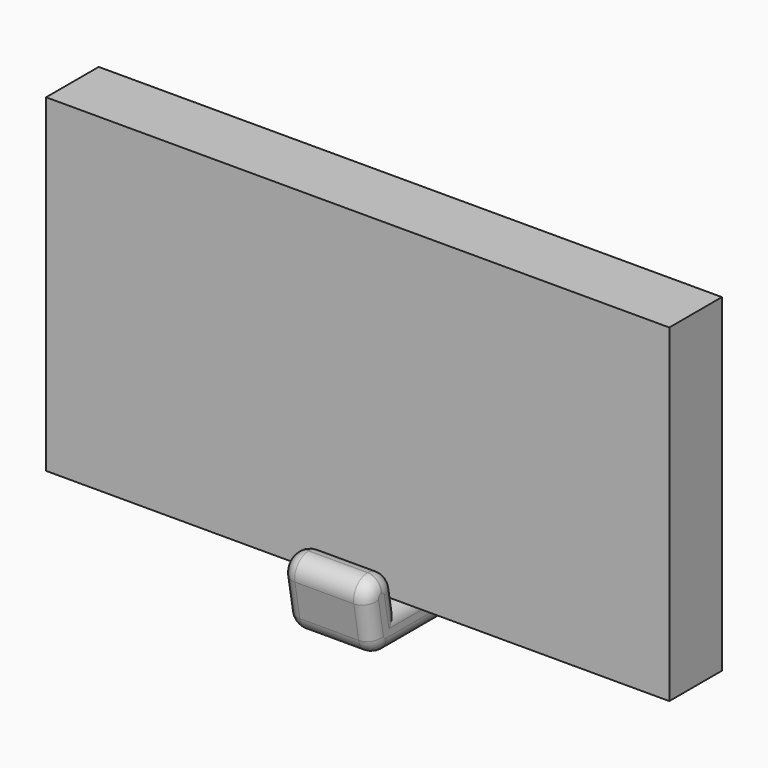
from build123d import *

# Parameters (mm, degrees)
F0_W          = 180
F0_H          = 95
F1_DEPTH      = 9.5
F3_W          = 10
F3_H          = 69.3333333333
F3_W_2        = 5
F3_H_2        = 10
F4_DEPTH      = 12.5
F5_T1_DEPTH   = 10.1542661189
F5_T3_DEPTH   = 65.3333333333
F5_T5_DEPTH   = 2
F5_T7_DEPTH   = 17
F5_T9_DEPTH   = 30.3474206258
F5_T11_DEPTH  = 70.3333333333
F5_T13_DEPTH  = 0.1519224699
F5_S17_W      = 4
F5_S17_H      = 4
F5_T18_DEPTH  = 4
F5_S23_W      = 4
F5_S23_H      = 4
F5_T24_DEPTH  = 4
F5_S29_W      = 4
F5_S29_H      = 4
F5_T30_DEPTH  = 4
F5_S35_W      = 4
F5_S35_H      = 4
F5_T36_DEPTH  = 4
F5_T42_DEPTH  = 31
F5_T47_DEPTH  = 31
F5_T50_ANGLE  = 100
F5_T52_ANGLE  = 80
F5_T54_ANGLE  = 90
F5_T56_ANGLE  = 80
F5_T60_DEPTH  = 15.958767963
F5_T63_ANGLE  = 100
F5_T65_ANGLE  = 80
F5_T67_ANGLE  = 90
F5_T69_ANGLE  = 80
F5_T73_DEPTH  = 15.958767963
F5_T79_DEPTH  = 75.3333333333
F5_T83_DEPTH  = 41
F5_T90_DEPTH  = 15.958767963
F5_T94_DEPTH  = 31
F5_T101_DEPTH = 75.3333333333
F5_T105_DEPTH = 41
F5_T112_DEPTH = 15.958767963
F5_T116_DEPTH = 31
F6_W          = 119.8909639199
F6_H          = 5
F7_DEPTH      = 5


# Not quite as in the source:
# - a fillet or chamfer that OpenCascade refuses, or shapes differently, is made with other operations: its cross-section is extruded or revolved along the edge and cut away or added


with BuildPart() as f1:
    # F0 (on Front) → F1 (new body, symmetric)
    with BuildSketch(Plane.XZ):
        Rectangle(F0_W, F0_H)
    extrude(amount=F1_DEPTH, both=True)


with BuildPart() as f4:
    # F3 (on Right) → F4 (new body, symmetric)
    with BuildSketch(Plane.YZ):
        with Locations((15.5, -13.8333333333)):
            Rectangle(F3_W, F3_H)
        with Locations((15.5, 10.8333333333)):
            Rectangle(F3_W_2, F3_H_2, mode=Mode.SUBTRACT)
        with BuildLine():
            Line((20.5, -53.5), (20.5, -48.5))
            Line((20.5, -48.5), (10.5, -48.5))
            Line((10.5, -48.5), (-10.5, -48.5))
            Line((-10.5, -48.5), (-8.7367301929, -58.5))
            Line((-8.7367301929, -58.5), (15.5, -58.5))
            ThreePointArc((15.5, -58.5), (19.0355339059, -57.0355339059), (20.5, -53.5))
        make_face()
        Polygon((-8.7367301929, -58.5), (-10.5, -48.5), (-10.5, -58.5), align=None)
        with BuildLine():
            Line((-10.5, -58.5), (-10.5, -48.5))
            Line((-10.5, -48.5), (-11.5347291979, -42.6317591117))
            ThreePointArc((-11.5347291979, -42.6317591117), (-13.2448299145, -39.6697777844), (-16.458767963, -38.5))
            Line((-16.458767963, -38.5), (-16.6106904328, -38.5))
            ThreePointArc((-16.6106904328, -38.5), (-20.4409126484, -40.2860619516), (-21.5347291979, -44.3682408883))
            Line((-21.5347291979, -44.3682408883), (-19.7714593908, -54.3682408883))
            ThreePointArc((-19.7714593908, -54.3682408883), (-18.0613586742, -57.3302222156), (-14.8474206258, -58.5))
            Line((-14.8474206258, -58.5), (-10.5, -58.5))
        make_face()
    extrude(amount=F4_DEPTH, both=True)

    # F5: fillet of radius 4 on 10 edges, made by hand

    # F5_s2 → F5_t1 (cut)
    with BuildSketch(Plane(origin=(0, 6.9380645139, -39.3477191408), x_dir=(1, 0, 0), z_dir=(0, 0.1736481777, -0.984807753))):
        with BuildLine():
            ThreePointArc((-8.5, 28.9120324497), (-11.3284271247, 27.7404595744), (-12.5, 24.9120324497))
            Line((-12.5, 24.9120324497), (-12.5, 28.9120324497))
            Line((-12.5, 28.9120324497), (-8.5, 28.9120324497))
        make_face()
        with BuildLine():
            ThreePointArc((8.5, 28.9120324497), (11.3284271247, 27.7404595744), (12.5, 24.9120324497))
            Line((12.5, 24.9120324497), (12.5, 28.9120324497))
            Line((12.5, 28.9120324497), (8.5, 28.9120324497))
        make_face()
    extrude(amount=F5_T1_DEPTH, mode=Mode.SUBTRACT)

    # F5_s4 → F5_t3 (cut)
    with BuildSketch(Plane.XY.offset(-48.5)):
        with BuildLine():
            ThreePointArc((8.5, 10.5), (11.3284271247, 11.6715728753), (12.5, 14.5))
            Line((12.5, 14.5), (12.5, 10.5))
            Line((12.5, 10.5), (8.5, 10.5))
        make_face()
        with BuildLine():
            ThreePointArc((-8.5, 10.5), (-11.3284271247, 11.6715728753), (-12.5, 14.5))
            Line((-12.5, 14.5), (-12.5, 10.5))
            Line((-12.5, 10.5), (-8.5, 10.5))
        make_face()
    extrude(amount=F5_T3_DEPTH, mode=Mode.SUBTRACT)

    # F5_s6 → F5_t5 (cut)
    with BuildSketch(Plane.XZ.offset(-16.5)):
        with BuildLine():
            ThreePointArc((-8.5, 20.8333333333), (-11.3284271247, 19.6617604581), (-12.5, 16.8333333333))
            Line((-12.5, 16.8333333333), (-12.5, 20.8333333333))
            Line((-12.5, 20.8333333333), (-8.5, 20.8333333333))
        make_face()
        with BuildLine():
            ThreePointArc((8.5, 20.8333333333), (11.3284271247, 19.6617604581), (12.5, 16.8333333333))
            Line((12.5, 16.8333333333), (12.5, 20.8333333333))
            Line((12.5, 20.8333333333), (8.5, 20.8333333333))
        make_face()
    extrude(amount=F5_T5_DEPTH, mode=Mode.SUBTRACT)

    # F5_s8 → F5_t7 (cut)
    with BuildSketch(Plane.YZ.offset(-8.5)):
        with BuildLine():
            ThreePointArc((10.5, 16.8333333333), (11.6715728753, 19.6617604581), (14.5, 20.8333333333))
            Line((14.5, 20.8333333333), (10.5, 20.8333333333))
            Line((10.5, 20.8333333333), (10.5, 16.8333333333))
        make_face()
        with BuildLine():
            ThreePointArc((16.5, 20.8333333333), (19.3284271247, 19.6617604581), (20.5, 16.8333333333))
            Line((20.5, 16.8333333333), (20.5, 20.8333333333))
            Line((20.5, 20.8333333333), (16.5, 20.8333333333))
        make_face()
    extrude(amount=F5_T7_DEPTH, mode=Mode.SUBTRACT)

    # F5_s10 → F5_t9 (cut)
    with BuildSketch(Plane.XZ.offset(-15.5)):
        with BuildLine():
            ThreePointArc((8.5, -58.5), (11.3284271247, -57.3284271247), (12.5, -54.5))
            Line((12.5, -54.5), (12.5, -58.5))
            Line((12.5, -58.5), (8.5, -58.5))
        make_face()
        with BuildLine():
            ThreePointArc((-8.5, -58.5), (-11.3284271247, -57.3284271247), (-12.5, -54.5))
            Line((-12.5, -54.5), (-12.5, -58.5))
            Line((-12.5, -58.5), (-8.5, -58.5))
        make_face()
    extrude(amount=F5_T9_DEPTH, mode=Mode.SUBTRACT)

    # F5_s12 → F5_t11 (cut)
    with BuildSketch(Plane.XY.offset(-53.5)):
        with BuildLine():
            ThreePointArc((8.5, 20.5), (11.3284271247, 19.3284271247), (12.5, 16.5))
            Line((12.5, 16.5), (12.5, 20.5))
            Line((12.5, 20.5), (8.5, 20.5))
        make_face()
        with BuildLine():
            ThreePointArc((-8.5, 20.5), (-11.3284271247, 19.3284271247), (-12.5, 16.5))
            Line((-12.5, 16.5), (-12.5, 20.5))
            Line((-12.5, 20.5), (-8.5, 20.5))
        make_face()
    extrude(amount=F5_T11_DEPTH, mode=Mode.SUBTRACT)

    # F5_s14 → F5_t13 (cut)
    with BuildSketch(Plane.XZ.offset(16.458767963)):
        with BuildLine():
            ThreePointArc((8.5, -38.5), (11.3284271247, -39.6715728753), (12.5, -42.5))
            Line((12.5, -42.5), (12.5, -38.5))
            Line((12.5, -38.5), (8.5, -38.5))
        make_face()
        with BuildLine():
            ThreePointArc((-8.5, -38.5), (-11.3284271247, -39.6715728753), (-12.5, -42.5))
            Line((-12.5, -42.5), (-12.5, -38.5))
            Line((-12.5, -38.5), (-8.5, -38.5))
        make_face()
    extrude(amount=F5_T13_DEPTH, mode=Mode.SUBTRACT)


with BuildPart() as f5_tool16:
    # F5_s17 → F5_t18 (new body)
    with BuildSketch(Plane.XZ.offset(-14.5)):
        with Locations((10.5, 18.8333333333)):
            Rectangle(F5_S17_W, F5_S17_H)
    extrude(amount=F5_T18_DEPTH)

    # F5_s19 → F5_t20 (revolve, cut)
    with BuildSketch(Plane(origin=(8.5, 14.5, 16.8333333333), x_dir=(-0.7071067812, 0, -0.7071067812), z_dir=(-0.7071067812, 0, 0.7071067812))):
        with BuildLine():
            ThreePointArc((0, -4), (4, 0), (0, 4))
            Line((0, 4), (0, -4))
        make_face()
    revolve(axis=Axis((8.5, 14.5, 16.8333333333), (0, -1, 0)), mode=Mode.SUBTRACT)


with BuildPart() as f4_1:
    add(f4.part)

    # F5_t15: cut F5_tool16
    add(f5_tool16.part, mode=Mode.SUBTRACT)


with BuildPart() as f5_tool22:
    # F5_s23 → F5_t24 (new body)
    with BuildSketch(Plane.XZ.offset(-14.5)):
        with Locations((-10.5, 18.8333333333)):
            Rectangle(F5_S23_W, F5_S23_H)
    extrude(amount=F5_T24_DEPTH)

    # F5_s25 → F5_t26 (revolve, cut)
    with BuildSketch(Plane(origin=(-8.5, 14.5, 16.8333333333), x_dir=(0.7071067812, 0, -0.7071067812), z_dir=(-0.7071067812, 0, -0.7071067812))):
        with BuildLine():
            ThreePointArc((0, -4), (4, 0), (0, 4))
            Line((0, 4), (0, -4))
        make_face()
    revolve(axis=Axis((-8.5, 14.5, 16.8333333333), (0, -1, 0)), mode=Mode.SUBTRACT)


with BuildPart() as f4_2:
    add(f4_1.part)

    # F5_t21: cut F5_tool22
    add(f5_tool22.part, mode=Mode.SUBTRACT)


with BuildPart() as f5_tool28:
    # F5_s29 → F5_t30 (new body)
    with BuildSketch(Plane.XY.offset(16.8333333333)):
        with Locations((-10.5, 18.5)):
            Rectangle(F5_S29_W, F5_S29_H)
    extrude(amount=F5_T30_DEPTH)

    # F5_s31 → F5_t32 (revolve, cut)
    with BuildSketch(Plane(origin=(-8.5, 16.5, 16.8333333333), x_dir=(0.7071067812, -0.7071067812, 0), z_dir=(-0.7071067812, -0.7071067812, 0))):
        with BuildLine():
            ThreePointArc((0, -4), (4, 0), (0, 4))
            Line((0, 4), (0, -4))
        make_face()
    revolve(axis=Axis((-8.5, 16.5, 16.8333333333), (0, 0, 1)), mode=Mode.SUBTRACT)


with BuildPart() as f4_3:
    add(f4_2.part)

    # F5_t27: cut F5_tool28
    add(f5_tool28.part, mode=Mode.SUBTRACT)


with BuildPart() as f5_tool34:
    # F5_s35 → F5_t36 (new body)
    with BuildSketch(Plane.XY.offset(16.8333333333)):
        with Locations((10.5, 18.5)):
            Rectangle(F5_S35_W, F5_S35_H)
    extrude(amount=F5_T36_DEPTH)

    # F5_s37 → F5_t38 (revolve, cut)
    with BuildSketch(Plane(origin=(8.5, 16.5, 16.8333333333), x_dir=(-0.7071067812, -0.7071067812, 0), z_dir=(-0.7071067812, 0.7071067812, 0))):
        with BuildLine():
            ThreePointArc((0, -4), (4, 0), (0, 4))
            Line((0, 4), (0, -4))
        make_face()
    revolve(axis=Axis((8.5, 16.5, 16.8333333333), (0, 0, 1)), mode=Mode.SUBTRACT)


with BuildPart() as f4_4:
    add(f4_3.part)

    # F5_t33: cut F5_tool34
    add(f5_tool34.part, mode=Mode.SUBTRACT)


with BuildPart() as f5_tool40:
    # F5_s41 → F5_t42 (new body)
    with BuildSketch(Plane.XZ.offset(-10.5)):
        with BuildLine():
            ThreePointArc((12.5, -52.5), (11.3284271247, -49.6715728753), (8.5, -48.5))
            Line((8.5, -48.5), (12.5, -48.5))
            Line((12.5, -48.5), (12.5, -52.5))
        make_face()
    extrude(amount=F5_T42_DEPTH)

    split(bisect_by=Plane(origin=(0, -18.4773747348, -3.2580596984), x_dir=(1, 0, 0), z_dir=(0, 0.984807753, 0.1736481777)), keep=Keep.TOP)


with BuildPart() as f4_5:
    add(f4_4.part)

    # F5_t39: cut F5_tool40
    add(f5_tool40.part, mode=Mode.SUBTRACT)


with BuildPart() as f5_tool45:
    # F5_s46 → F5_t47 (new body)
    with BuildSketch(Plane.XZ.offset(-10.5)):
        with BuildLine():
            ThreePointArc((-8.5, -48.5), (-11.3284271247, -49.6715728753), (-12.5, -52.5))
            Line((-12.5, -52.5), (-12.5, -48.5))
            Line((-12.5, -48.5), (-8.5, -48.5))
        make_face()
    extrude(amount=F5_T47_DEPTH)

    split(bisect_by=Plane(origin=(0, -18.4773747348, -3.2580596984), x_dir=(1, 0, 0), z_dir=(0, 0.984807753, 0.1736481777)), keep=Keep.TOP)


with BuildPart() as f4_6:
    add(f4_5.part)

    # F5_t44: cut F5_tool45
    add(f5_tool45.part, mode=Mode.SUBTRACT)

    # F5_s49 → F5_t50 (revolve, cut)
    with BuildSketch(Plane.XZ.offset(16.6106904328)):
        with BuildLine():
            ThreePointArc((8.5, -38.5), (11.3284271247, -39.6715728753), (12.5, -42.5))
            Line((12.5, -42.5), (12.5, -38.5))
            Line((12.5, -38.5), (8.5, -38.5))
        make_face()
    revolve(axis=Axis((12.5, -16.6106904328, -43.5), (1, 0, 0)), revolution_arc=F5_T50_ANGLE, mode=Mode.SUBTRACT)

    # F5_s51 → F5_t52 (revolve, cut)
    with BuildSketch(Plane(origin=(0, 8.7013343209, -49.3477191408), x_dir=(1, 0, 0), z_dir=(0, -0.1736481777, 0.984807753))):
        with BuildLine():
            ThreePointArc((8.5, -28.9120324497), (11.3284271247, -27.7404595744), (12.5, -24.9120324497))
            Line((12.5, -24.9120324497), (12.5, -28.9120324497))
            Line((12.5, -28.9120324497), (8.5, -28.9120324497))
        make_face()
    revolve(axis=Axis((12.5, -14.8474206258, -53.5), (1, 0, 0)), revolution_arc=F5_T52_ANGLE, mode=Mode.SUBTRACT)

    # F5_s53 → F5_t54 (revolve, cut)
    with BuildSketch(Plane.XZ.offset(-15.5)):
        with BuildLine():
            ThreePointArc((8.5, -58.5), (11.3284271247, -57.3284271247), (12.5, -54.5))
            Line((12.5, -54.5), (12.5, -58.5))
            Line((12.5, -58.5), (8.5, -58.5))
        make_face()
    revolve(axis=Axis((12.5, 15.5, -53.5), (1, 0, 0)), revolution_arc=F5_T54_ANGLE, mode=Mode.SUBTRACT)

    # F5_s55 → F5_t56 (revolve, cut)
    with BuildSketch(Plane(origin=(0, 6.9426455369, -39.3736994133), x_dir=(1, 0, 0), z_dir=(0, 0.1736481777, -0.984807753))):
        with BuildLine():
            ThreePointArc((8.5, 18.7624180235), (11.3284271247, 19.9339908987), (12.5, 22.7624180235))
            Line((12.5, 22.7624180235), (12.5, 18.7624180235))
            Line((12.5, 18.7624180235), (8.5, 18.7624180235))
        make_face()
    revolve(axis=Axis((12.5, -16.458767963, -43.5), (1, 0, 0)), revolution_arc=F5_T56_ANGLE, mode=Mode.SUBTRACT)


with BuildPart() as f5_tool58:
    # F5_s59 → F5_t60 (new body)
    with BuildSketch(Plane(origin=(0, 9.7138565114, -55.0900178317), x_dir=(1, 0, 0), z_dir=(0, -0.1736481777, 0.984807753))):
        with BuildLine():
            ThreePointArc((8.5, -18.7624180235), (11.3284271247, -19.9339908987), (12.5, -22.7624180235))
            Line((12.5, -22.7624180235), (12.5, -18.7624180235))
            Line((12.5, -18.7624180235), (8.5, -18.7624180235))
        make_face()
    extrude(amount=F5_T60_DEPTH)

    split(bisect_by=Plane.XY.offset(-48.5), keep=Keep.TOP)


with BuildPart() as f4_7:
    add(f4_6.part)

    # F5_t57: cut F5_tool58
    add(f5_tool58.part, mode=Mode.SUBTRACT)

    # F5_s62 → F5_t63 (revolve, cut)
    with BuildSketch(Plane.XZ.offset(16.6106904328)):
        with BuildLine():
            ThreePointArc((-8.5, -38.5), (-11.3284271247, -39.6715728753), (-12.5, -42.5))
            Line((-12.5, -42.5), (-12.5, -38.5))
            Line((-12.5, -38.5), (-8.5, -38.5))
        make_face()
    revolve(axis=Axis((-12.5, -16.6106904328, -43.5), (1, 0, 0)), revolution_arc=F5_T63_ANGLE, mode=Mode.SUBTRACT)

    # F5_s64 → F5_t65 (revolve, cut)
    with BuildSketch(Plane(origin=(0, 8.7013343209, -49.3477191408), x_dir=(1, 0, 0), z_dir=(0, -0.1736481777, 0.984807753))):
        with BuildLine():
            ThreePointArc((-8.5, -28.9120324497), (-11.3284271247, -27.7404595744), (-12.5, -24.9120324497))
            Line((-12.5, -24.9120324497), (-12.5, -28.9120324497))
            Line((-12.5, -28.9120324497), (-8.5, -28.9120324497))
        make_face()
    revolve(axis=Axis((-12.5, -14.8474206258, -53.5), (1, 0, 0)), revolution_arc=F5_T65_ANGLE, mode=Mode.SUBTRACT)

    # F5_s66 → F5_t67 (revolve, cut)
    with BuildSketch(Plane.XZ.offset(-15.5)):
        with BuildLine():
            ThreePointArc((-8.5, -58.5), (-11.3284271247, -57.3284271247), (-12.5, -54.5))
            Line((-12.5, -54.5), (-12.5, -58.5))
            Line((-12.5, -58.5), (-8.5, -58.5))
        make_face()
    revolve(axis=Axis((-12.5, 15.5, -53.5), (1, 0, 0)), revolution_arc=F5_T67_ANGLE, mode=Mode.SUBTRACT)

    # F5_s68 → F5_t69 (revolve, cut)
    with BuildSketch(Plane(origin=(0, 6.9426455369, -39.3736994133), x_dir=(1, 0, 0), z_dir=(0, 0.1736481777, -0.984807753))):
        with BuildLine():
            ThreePointArc((-8.5, 18.7624180235), (-11.3284271247, 19.9339908987), (-12.5, 22.7624180235))
            Line((-12.5, 22.7624180235), (-12.5, 18.7624180235))
            Line((-12.5, 18.7624180235), (-8.5, 18.7624180235))
        make_face()
    revolve(axis=Axis((-12.5, -16.458767963, -43.5), (1, 0, 0)), revolution_arc=F5_T69_ANGLE, mode=Mode.SUBTRACT)


with BuildPart() as f5_tool71:
    # F5_s72 → F5_t73 (new body)
    with BuildSketch(Plane(origin=(0, 9.7138565114, -55.0900178317), x_dir=(1, 0, 0), z_dir=(0, -0.1736481777, 0.984807753))):
        with BuildLine():
            ThreePointArc((-8.5, -18.7624180235), (-11.3284271247, -19.9339908987), (-12.5, -22.7624180235))
            Line((-12.5, -22.7624180235), (-12.5, -18.7624180235))
            Line((-12.5, -18.7624180235), (-8.5, -18.7624180235))
        make_face()
    extrude(amount=F5_T73_DEPTH)

    split(bisect_by=Plane.XY.offset(-48.5), keep=Keep.TOP)


with BuildPart() as f4_8:
    add(f4_7.part)

    # F5_t70: cut F5_tool71
    add(f5_tool71.part, mode=Mode.SUBTRACT)


with BuildPart() as f5_tool77:
    # F5_s78 → F5_t79 (new body)
    with BuildSketch(Plane.XY.offset(16.8333333333)):
        with BuildLine():
            ThreePointArc((8.5, 10.5), (11.3284271247, 11.6715728753), (12.5, 14.5))
            Line((12.5, 14.5), (12.5, 10.5))
            Line((12.5, 10.5), (8.5, 10.5))
        make_face()
    extrude(amount=-F5_T79_DEPTH)

    split(bisect_by=Plane.XY.offset(-48.5), keep=Keep.BOTTOM)


with BuildPart() as f5_tool81:
    # F5_s82 → F5_t83 (new body)
    with BuildSketch(Plane.XZ.offset(-20.5)):
        with BuildLine():
            ThreePointArc((12.5, -52.5), (11.3284271247, -49.6715728753), (8.5, -48.5))
            Line((8.5, -48.5), (12.5, -48.5))
            Line((12.5, -48.5), (12.5, -52.5))
        make_face()
    extrude(amount=F5_T83_DEPTH)

    split(bisect_by=Plane.XZ.offset(-10.5), keep=Keep.BOTTOM)


with BuildPart() as f5_tool77_1:
    add(f5_tool77.part)

    # F5_t85: intersect F5_tool81
    add(f5_tool81.part, mode=Mode.INTERSECT)


with BuildPart() as f4_9:
    add(f4_8.part)

    # F5_t75: cut F5_tool77
    add(f5_tool77_1.part, mode=Mode.SUBTRACT)


with BuildPart() as f5_tool88:
    # F5_s89 → F5_t90 (new body)
    with BuildSketch(Plane(origin=(0, 9.7138565114, -55.0900178317), x_dir=(1, 0, 0), z_dir=(0, -0.1736481777, 0.984807753))):
        with BuildLine():
            ThreePointArc((8.5, -18.7624180235), (11.3284271247, -19.9339908987), (12.5, -22.7624180235))
            Line((12.5, -22.7624180235), (12.5, -18.7624180235))
            Line((12.5, -18.7624180235), (8.5, -18.7624180235))
        make_face()
    extrude(amount=F5_T90_DEPTH)

    split(bisect_by=Plane.XY.offset(-48.5), keep=Keep.BOTTOM)


with BuildPart() as f5_tool92:
    # F5_s93 → F5_t94 (new body)
    with BuildSketch(Plane.XZ.offset(-10.5)):
        with BuildLine():
            ThreePointArc((12.5, -52.5), (11.3284271247, -49.6715728753), (8.5, -48.5))
            Line((8.5, -48.5), (12.5, -48.5))
            Line((12.5, -48.5), (12.5, -52.5))
        make_face()
    extrude(amount=F5_T94_DEPTH)

    split(bisect_by=Plane(origin=(0, -18.4773747348, -3.2580596984), x_dir=(1, 0, 0), z_dir=(0, -0.984807753, -0.1736481777)), keep=Keep.TOP)


with BuildPart() as f5_tool88_1:
    add(f5_tool88.part)

    # F5_t96: intersect F5_tool92
    add(f5_tool92.part, mode=Mode.INTERSECT)


with BuildPart() as f4_10:
    add(f4_9.part)

    # F5_t86: cut F5_tool88
    add(f5_tool88_1.part, mode=Mode.SUBTRACT)


with BuildPart() as f5_tool99:
    # F5_s100 → F5_t101 (new body)
    with BuildSketch(Plane.XY.offset(16.8333333333)):
        with BuildLine():
            ThreePointArc((-8.5, 10.5), (-11.3284271247, 11.6715728753), (-12.5, 14.5))
            Line((-12.5, 14.5), (-12.5, 10.5))
            Line((-12.5, 10.5), (-8.5, 10.5))
        make_face()
    extrude(amount=-F5_T101_DEPTH)

    split(bisect_by=Plane.XY.offset(-48.5), keep=Keep.BOTTOM)


with BuildPart() as f5_tool103:
    # F5_s104 → F5_t105 (new body)
    with BuildSketch(Plane.XZ.offset(-20.5)):
        with BuildLine():
            ThreePointArc((-8.5, -48.5), (-11.3284271247, -49.6715728753), (-12.5, -52.5))
            Line((-12.5, -52.5), (-12.5, -48.5))
            Line((-12.5, -48.5), (-8.5, -48.5))
        make_face()
    extrude(amount=F5_T105_DEPTH)

    split(bisect_by=Plane.XZ.offset(-10.5), keep=Keep.BOTTOM)


with BuildPart() as f5_tool99_1:
    add(f5_tool99.part)

    # F5_t107: intersect F5_tool103
    add(f5_tool103.part, mode=Mode.INTERSECT)


with BuildPart() as f4_11:
    add(f4_10.part)

    # F5_t97: cut F5_tool99
    add(f5_tool99_1.part, mode=Mode.SUBTRACT)


with BuildPart() as f5_tool110:
    # F5_s111 → F5_t112 (new body)
    with BuildSketch(Plane(origin=(0, 9.7138565114, -55.0900178317), x_dir=(1, 0, 0), z_dir=(0, -0.1736481777, 0.984807753))):
        with BuildLine():
            ThreePointArc((-8.5, -18.7624180235), (-11.3284271247, -19.9339908987), (-12.5, -22.7624180235))
            Line((-12.5, -22.7624180235), (-12.5, -18.7624180235))
            Line((-12.5, -18.7624180235), (-8.5, -18.7624180235))
        make_face()
    extrude(amount=F5_T112_DEPTH)

    split(bisect_by=Plane.XY.offset(-48.5), keep=Keep.BOTTOM)


with BuildPart() as f5_tool114:
    # F5_s115 → F5_t116 (new body)
    with BuildSketch(Plane.XZ.offset(-10.5)):
        with BuildLine():
            ThreePointArc((-8.5, -48.5), (-11.3284271247, -49.6715728753), (-12.5, -52.5))
            Line((-12.5, -52.5), (-12.5, -48.5))
            Line((-12.5, -48.5), (-8.5, -48.5))
        make_face()
    extrude(amount=F5_T116_DEPTH)

    split(bisect_by=Plane(origin=(0, -18.4773747348, -3.2580596984), x_dir=(1, 0, 0), z_dir=(0, -0.984807753, -0.1736481777)), keep=Keep.TOP)


with BuildPart() as f5_tool110_1:
    add(f5_tool110.part)

    # F5_t118: intersect F5_tool114
    add(f5_tool114.part, mode=Mode.INTERSECT)


with BuildPart() as f4_12:
    add(f4_11.part)

    # F5_t108: cut F5_tool110
    add(f5_tool110_1.part, mode=Mode.SUBTRACT)


with BuildPart() as f7:
    # F6 (on Top) → F7 (new body)
    with BuildSketch(Plane.XY):
        with Locations((-37.2533172926, 36.5193495899)):
            Rectangle(F6_W, F6_H)
        with BuildLine():
            Line((-97.1987992525, 34.0193495899), (-97.1987992525, 39.0193495899))
            ThreePointArc((-97.1987992525, 39.0193495899), (-112.1987992525, 24.0193495899), (-97.1987992525, 9.0193495899))
            ThreePointArc((-97.1987992525, 9.0193495899), (-94.6987992525, 11.5193495899), (-97.1987992525, 14.0193495899))
            ThreePointArc((-97.1987992525, 14.0193495899), (-107.1987992525, 24.0193495899), (-97.1987992525, 34.0193495899))
        make_face()
    extrude(amount=F7_DEPTH)


solid = Compound([f1.part, f4_12.part, f7.part])
